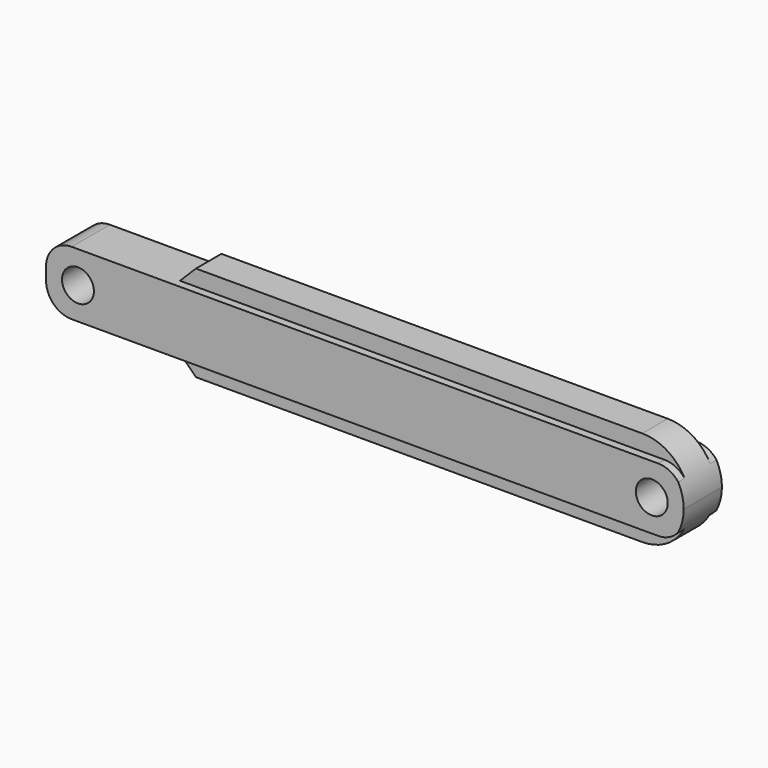
from build123d import *

# Parameters (mm, degrees)
F0_W          = 127
F0_H          = 12.7
F0_R          = 3.175
F1_DEPTH      = 9.525
F2_R          = 5.08
F5_W          = 101.6
F5_H          = 19.05
F6_DEPTH      = 3.175
F6_DEPTH_BACK = 3.175
F7_SIZE       = 3.17499
F8_R          = 9.52499


# Not quite as in the source:
# - a fillet or chamfer is up to 0.001 mm smaller than in the source, because OpenCascade refuses the exact size


with BuildPart() as f1:
    # F0 (on Front) → F1 (new body)
    with BuildSketch(Plane.XZ):
        Rectangle(F0_W, F0_H)
        with Locations((-57.15, 0)):
            Circle(F0_R, mode=Mode.SUBTRACT)
        with Locations((57.15, 0)):
            Circle(F0_R, mode=Mode.SUBTRACT)
    extrude(amount=F1_DEPTH)

    # F2
    f2_edges = [f1.edges().sort_by_distance(p)[0] for p in [
        (-63.5, -4.7625, 6.35),
        (-63.5, -4.7625, -6.35),
        (63.5, -4.7625, 6.35),
        (63.5, -4.7625, -6.35),
    ]]
    fillet(f2_edges, radius=F2_R)

    # F5 (on face) → F6 (join, two sides)
    with BuildSketch(Plane(origin=(0, -4.7625, 0), x_dir=(-1, 0, 0), z_dir=(0, 1, 0))) as f6_sk:
        with Locations((-12.7, 0)):
            Rectangle(F5_W, F5_H)
        with BuildLine():
            ThreePointArc((-57.1005828679, 4.1822632775), (-52.9233760572, 0.0930895553), (-57.0553988218, -4.0417364798))
            ThreePointArc((-57.0553988218, -4.0417364798), (-61.2736674525, 0.0472116417), (-57.1005828679, 4.1822632775))
        make_face(mode=Mode.SUBTRACT)
    extrude(amount=F6_DEPTH)
    extrude(f6_sk.sketch, amount=-F6_DEPTH_BACK)

    # F7 (size 3.175 in the source; OpenCascade refuses exactly that, so slightly less here)
    f7_edges = [f1.edges().sort_by_distance(p)[0] for p in [
        (-38.1, -4.7625, 9.525),
        (-38.1, -4.7625, -9.525),
    ]]
    chamfer(f7_edges, length=F7_SIZE)

    # F8 (radius 9.525 in the source; OpenCascade refuses exactly that, so slightly less here)
    f8_edges = [f1.edges().sort_by_distance(p)[0] for p in [
        (63.5, -4.7625, 9.525),
        (63.5, -4.7625, -9.525),
    ]]
    fillet(f8_edges, radius=F8_R)


solid = f1.part
